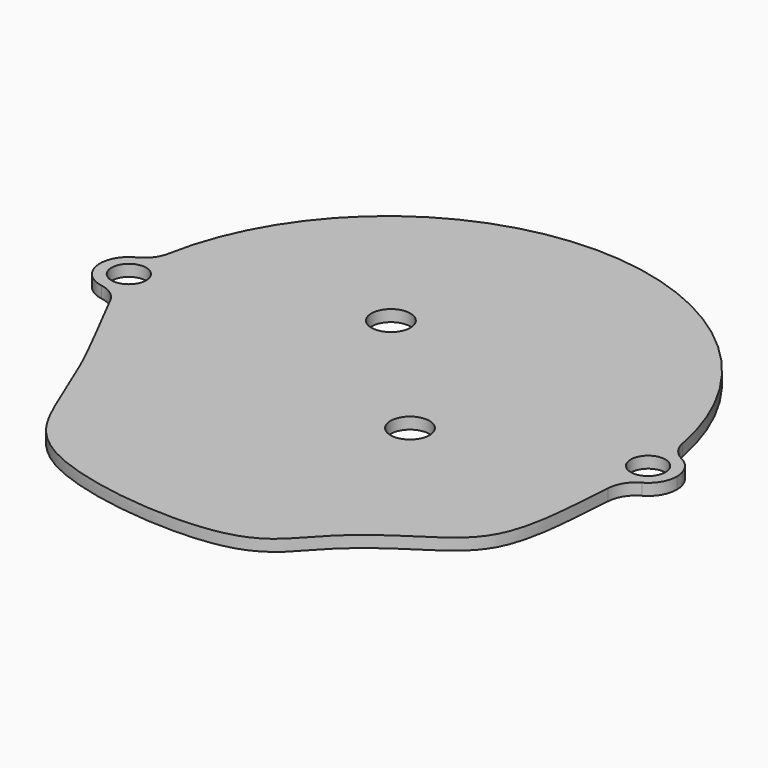
from build123d import *

# Parameters (mm, degrees)
F1_DEPTH = 2
F2_D     = 6
F2_DEPTH = 15
F2_TIP   = 1.8025818571
F3_R     = 5
F5_D     = 6.7564
F5_DEPTH = 15
F5_TIP   = 2.0298273432


# Not quite as in the source:
# - a feature names something its author has since deleted; it is built from what else it names


with BuildPart() as f1:
    # F0 (on Top) → F1 (new body)
    with BuildSketch(Plane.XY):
        with BuildLine():
            ThreePointArc((-47.3500001504, 5), (-43.8144662445, 3.5355339059), (-42.3500001504, 0))
            ThreePointArc((-42.3500001504, 0), (-43.3356192267, -2.9807290717), (-45.90389847, -4.7863127698))
            add(Edge.make_bspline(
                [(42.6499998496, -5), (42.5289111679, -9.8051674108), (42.0457129188, -14.7439877194), (40.7461175667, -30.1142148215), (29.7360021605, -36.317695818), (20.6555192756, -43.1714469496), (13.3678454871, -54.4108770899), (-23.6320989357, -50.5771015914), (-30.9587242182, -37.5079780838), (-35.7625076425, -23.9287004601), (-42.056342597, -12.5684016954), (-45.90389847, -4.7863127698)],
                knots=[0, 0, 0, 0, 0.0930383933, 0.1976366945, 0.2961687037, 0.3908471592, 0.4898375832, 0.6543651822, 0.7604357564, 0.8654232461, 1, 1, 1, 1], degree=3))
            ThreePointArc((42.6499998496, -5), (37.6499998496, 0), (42.6499998496, 5))
            ThreePointArc((42.6499998496, 5), (-2.3500001504, 45.0609898081), (-47.3500001504, 5))
        make_face()
        with BuildLine():
            ThreePointArc((-45.90389847, -4.7863127698), (-43.3356192267, -2.9807290717), (-42.3500001504, 0))
            ThreePointArc((-42.3500001504, 0), (-43.8144662445, 3.5355339059), (-47.3500001504, 5))
            ThreePointArc((-47.3500001504, 5), (-52.2962898634, -0.730902234), (-45.90389847, -4.7863127698))
        make_face()
        with BuildLine():
            ThreePointArc((47.6499998496, 0), (46.1855337555, 3.5355339059), (42.6499998496, 5))
            ThreePointArc((42.6499998496, 5), (37.6499998496, 0), (42.6499998496, -5))
            ThreePointArc((42.6499998496, -5), (46.1855337555, -3.5355339059), (47.6499998496, 0))
        make_face()
    extrude(amount=F1_DEPTH)

    # F2
    with Locations(Plane(origin=(0, 0, 0), x_dir=(1, 0, 0), z_dir=(0, 0, -1))):
        with Locations((-47.3500001504, 0), (42.6499998496, 0)):
            Hole(F2_D / 2, depth=F2_DEPTH)
            with Locations((0, 0, -(F2_DEPTH + F2_TIP / 2))):  # 118° drill point
                Cone(0, F2_D / 2, F2_TIP, mode=Mode.SUBTRACT)

    # F3
    f3_edges = [f1.edges().sort_by_distance(p)[0] for p in [
        (-47.35, 5, 1),
        (-45.903898, -4.786313, 1),
        (42.65, 5, 1),
        (42.65, -5, 1),
    ]]
    fillet(f3_edges, radius=F3_R)

    # F5
    with Locations(Plane.XY.offset(2)):
        with Locations((-11.1333334838, 11.5044798038), (10.5664664879, -11.4821037278)):
            Hole(F5_D / 2, depth=F5_DEPTH)
            with Locations((0, 0, -(F5_DEPTH + F5_TIP / 2))):  # 118° drill point
                Cone(0, F5_D / 2, F5_TIP, mode=Mode.SUBTRACT)


solid = f1.part
